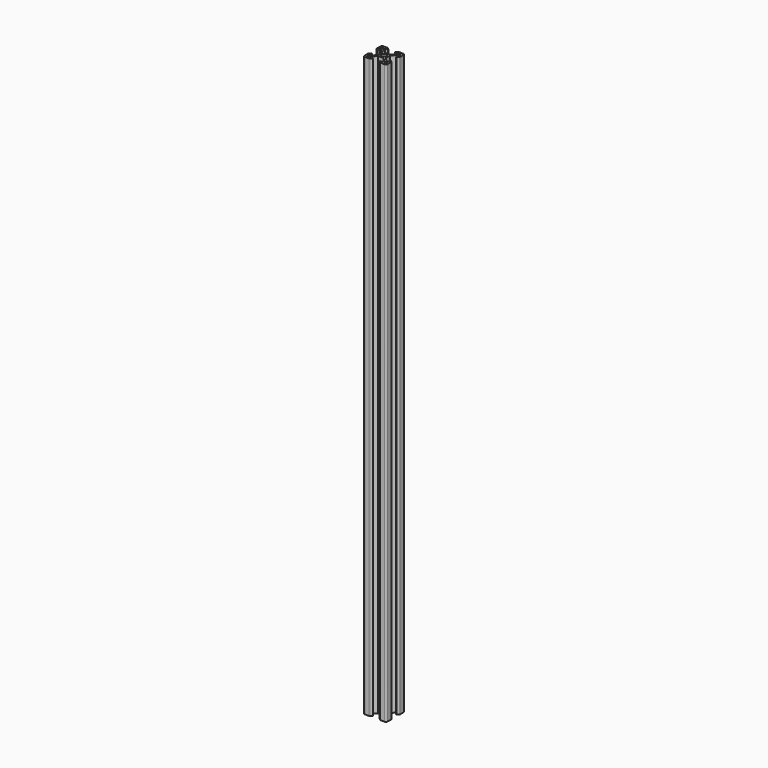
from build123d import *

# Parameters (mm, degrees)
F0_R     = 2.1
F1_DEPTH = 500


# Not quite as in the source:
# - ends of sketch curves that miss each other by under 0.0002 mm in the source are joined


with BuildPart() as f1:
    # F0 (on Top) → F1 (new body)
    with BuildSketch(Plane.XY):
        with BuildLine():
            Line((-8.2, 5.5), (-6.56066, 5.5))
            Line((-6.56066, 5.5), (-3.4, 2.33934))
            Line((-3.4, 2.33934), (-3.4, -2.33934))
            Line((-3.4, -2.33934), (-6.56066, -5.5))
            Line((-6.56066, -5.5), (-8.2, -5.5))
            Line((-8.2, -5.5), (-8.2, -2.89))
            Line((-8.2, -2.89), (-8.31, -2.89))
            Line((-8.31, -2.89), (-9.768614, -4.348614))
            ThreePointArc((-9.768614, -4.348614), (-9.9398646954, -4.6049087618), (-10, -4.907229))
            Line((-10, -4.907229), (-10, -8.5))
            ThreePointArc((-10, -8.5), (-9.5606601718, -9.5606601718), (-8.5, -10))
            Line((-8.5, -10), (-4.907229, -10))
            ThreePointArc((-4.907229, -10), (-4.6049087618, -9.9398646954), (-4.3486141429, -9.7686138571))
            Line((-4.3486141429, -9.7686138571), (-2.89, -8.31))
            Line((-2.89, -8.31), (-2.89, -8.2))
            Line((-2.89, -8.2), (-5.5, -8.2))
            Line((-5.5, -8.2), (-5.5, -6.56066))
            Line((-5.5, -6.56066), (-2.33934, -3.4))
            Line((-2.33934, -3.4), (2.33934, -3.4))
            Line((2.33934, -3.4), (5.5, -6.56066))
            Line((5.5, -6.56066), (5.5, -8.2))
            Line((5.5, -8.2), (2.89, -8.2))
            Line((2.89, -8.2), (2.89, -8.31))
            Line((2.89, -8.31), (4.348614, -9.768614))
            ThreePointArc((4.348614, -9.768614), (4.6049087618, -9.9398646954), (4.907229, -10))
            Line((4.907229, -10), (8.5, -10))
            ThreePointArc((8.5, -10), (9.5606601718, -9.5606601718), (10, -8.5))
            Line((10, -8.5), (10, -4.907229))
            ThreePointArc((10, -4.907229), (9.9398646954, -4.6049087618), (9.7686138571, -4.3486141429))
            Line((9.7686138571, -4.3486141429), (8.31, -2.89))
            Line((8.31, -2.89), (8.2, -2.89))
            Line((8.2, -2.89), (8.2, -5.5))
            Line((8.2, -5.5), (6.56066, -5.5))
            Line((6.56066, -5.5), (3.4, -2.33934))
            Line((3.4, -2.33934), (3.4, 2.33934))
            Line((3.4, 2.33934), (6.56066, 5.5))
            Line((6.56066, 5.5), (8.2, 5.5))
            Line((8.2, 5.5), (8.2, 2.89))
            Line((8.2, 2.89), (8.31, 2.89))
            Line((8.31, 2.89), (9.768614, 4.348614))
            ThreePointArc((9.768614, 4.348614), (9.9398646954, 4.6049087618), (10, 4.907229))
            Line((10, 4.907229), (10, 8.5))
            ThreePointArc((10, 8.5), (9.5606601718, 9.5606601718), (8.5, 10))
            Line((8.5, 10), (4.907229, 10))
            ThreePointArc((4.907229, 10), (4.6049087618, 9.9398646954), (4.3486141429, 9.7686138571))
            Line((4.3486141429, 9.7686138571), (2.89, 8.31))
            Line((2.89, 8.31), (2.89, 8.2))
            Line((2.89, 8.2), (5.5, 8.2))
            Line((5.5, 8.2), (5.5, 6.56066))
            Line((5.5, 6.56066), (2.33934, 3.4))
            Line((2.33934, 3.4), (-2.33934, 3.4))
            Line((-2.33934, 3.4), (-5.5, 6.56066))
            Line((-5.5, 6.56066), (-5.5, 8.2))
            Line((-5.5, 8.2), (-2.89, 8.2))
            Line((-2.89, 8.2), (-2.89, 8.31))
            Line((-2.89, 8.31), (-4.348614, 9.768614))
            ThreePointArc((-4.348614, 9.768614), (-4.6049087618, 9.9398646954), (-4.907229, 10))
            Line((-4.907229, 10), (-8.5, 10))
            ThreePointArc((-8.5, 10), (-9.5606601718, 9.5606601718), (-10, 8.5))
            Line((-10, 8.5), (-10, 4.907229))
            ThreePointArc((-10, 4.907229), (-9.9398646954, 4.6049087618), (-9.7686138571, 4.3486141429))
            Line((-9.7686138571, 4.3486141429), (-8.31, 2.89))
            Line((-8.31, 2.89), (-8.2, 2.89))
            Line((-8.2, 2.89), (-8.2, 5.5))
        make_face()
        Polygon((-6.57, -8.2), (-8.2, -8.2), (-8.2, -6.57), (-7.66, -6.57), (-6.57, -7.66), align=None, mode=Mode.SUBTRACT)
        Polygon((6.57, -7.66), (7.66, -6.57), (8.2, -6.57), (8.2, -8.2), (6.57, -8.2), align=None, mode=Mode.SUBTRACT)
        Polygon((-6.57, 7.66), (-7.66, 6.57), (-8.2, 6.57), (-8.2, 8.2), (-6.57, 8.2), align=None, mode=Mode.SUBTRACT)
        Circle(F0_R, mode=Mode.SUBTRACT)
        Polygon((6.57, 8.2), (8.2, 8.2), (8.2, 6.57), (7.66, 6.57), (6.57, 7.66), align=None, mode=Mode.SUBTRACT)
    extrude(amount=F1_DEPTH)


solid = f1.part
